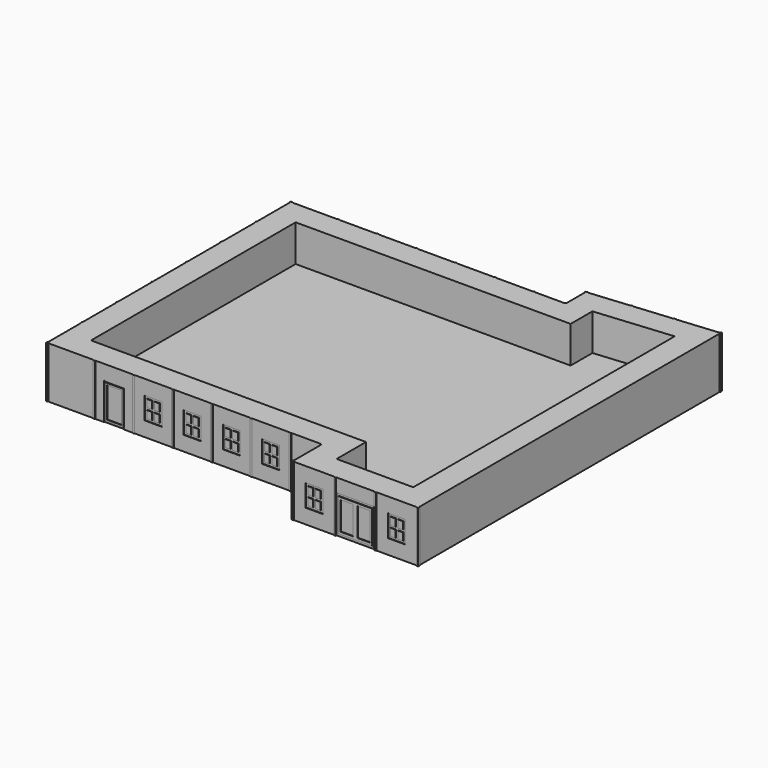
from build123d import *

# Parameters (mm, degrees)
F1_DEPTH  = 42
F3_DEPTH  = 30
F4_W      = 1.6
F4_H      = 42
F4_W_2    = 0.8
F6_W      = 1.6
F6_H      = 42
F13_DEPTH = 0.4
F5_W      = 0.8
F5_H      = 42
F5_W_2    = 1.6
F8_W      = 1.6
F8_H      = 42
F10_W     = 0.8
F10_H     = 42
F10_W_2   = 1.6
F14_DEPTH = 0.4
F7_W      = 0.4
F7_H      = 42
F7_W_2    = 1.2
F12_W     = 0.4368792842
F12_H     = 42
F12_W_2   = 1.1631207158
F12_W_3   = 0.3631207158
F15_DEPTH = 0.4
F9_W      = 1.6
F9_H      = 42
F9_W_2    = 0.8
F11_W     = 1.6
F11_H     = 42
F16_DEPTH = 0.4
F17_W     = 14.1428571429
F17_H     = 18
F17_W_2   = 4.1785714286
F17_H_2   = 6.1071428571
F18_W     = 14.1428571429
F18_H     = 18
F18_W_2   = 4.1785714286
F18_H_2   = 6.1071428571
F19_W     = 14.1428571429
F19_H     = 18
F19_W_2   = 4.1785714286
F19_H_2   = 6.1071428571
F20_DEPTH = 0.5
F21_W     = 17
F21_H     = 30
F21_W_2   = 15
F21_H_2   = 28
F21_W_3   = 12
F21_H_3   = 25
F22_DEPTH = 0.5
F23_W     = 31.4
F23_H     = 31
F23_W_2   = 27.4
F23_H_2   = 27
F23_W_3   = 10
F23_H_3   = 23
F24_DEPTH = 0.5
F25_W     = 14.1428571429
F25_H     = 18
F25_W_2   = 4.1785714286
F25_H_2   = 6.1071428571
F26_W     = 30.4
F26_H     = 31
F26_W_2   = 26.4
F26_H_2   = 27
F26_W_3   = 10
F26_H_3   = 23
F27_DEPTH = 0.5
F28_W     = 4.1785714286
F28_H     = 6.1071428571
F28_W_2   = 14.1428571429
F28_H_2   = 18
F29_DEPTH = 0.5


# Not quite as in the source:
# - a feature names something its author has since deleted; it is built from what else it names


with BuildPart() as f1:
    # F0 (on Top) → F1 (new body)
    with BuildSketch(Plane.XY):
        Polygon((-327.3, 108.1424002851), (-327.3, -140.8575997149), (-102.6, -140.8575997149), (-102.6, -170.8575997149), (0, -170.8575997149), (0, -140.8575997149), (0, 108.1424002851), (0, 138.1424002851), (-102.6, 128.6424002851), (-102.6, 108.1424002851), align=None)
    extrude(amount=F1_DEPTH)

    # F2 (on face) → F3 (cut)
    with BuildSketch(Plane.XY.offset(42)):
        Polygon((-20, 88.1424002851), (-20, 116.2049975252), (-82.6, 110.4087012289), (-82.6, 88.1424002851), (-307.3, 88.1424002851), (-307.3, -120.8575997149), (-82.6, -120.8575997149), (-82.6, -150.8575997149), (-20, -150.8575997149), (-20, -120.8575997149), align=None)
    extrude(amount=-F3_DEPTH, mode=Mode.SUBTRACT)

    # F4 (on face) + F6 (on face) → F13 (join)
    with BuildSketch(Plane.XZ.offset(140.8575997149)):
        with Locations((-288.375, 21)):
            Rectangle(F4_W, F4_H)
        with Locations((-256.375, 21)):
            Rectangle(F4_W, F4_H)
        with Locations((-224.375, 21)):
            Rectangle(F4_W, F4_H)
        with Locations((-192.375, 21)):
            Rectangle(F4_W, F4_H)
        with Locations((-160.375, 21)):
            Rectangle(F4_W, F4_H)
        with Locations((-128.375, 21)):
            Rectangle(F4_W, F4_H)
        with Locations((-103, 21)):
            Rectangle(F4_W_2, F4_H)
        with Locations((-326.9, 21)):
            Rectangle(F4_W, F4_H)
    with BuildSketch(Plane.XZ.offset(170.8575997149)):
        with Locations((-102.2, 21)):
            Rectangle(F6_W, F6_H)
        with Locations((-0.4, 21)):
            Rectangle(F6_W, F6_H)
        with Locations((-34.8, 21)):
            Rectangle(F6_W, F6_H)
        with Locations((-67.8, 21)):
            Rectangle(F6_W, F6_H)
    extrude(amount=F13_DEPTH)

    # F5 (on face) + F8 (on face) + F10 (on face) → F14 (join)
    with BuildSketch(Plane(origin=(-102.6, 0, 0), x_dir=(0, -1, 0), z_dir=(-1, 0, 0))):
        with Locations((141.2575997149, 21)):
            Rectangle(F5_W, F5_H)
        with Locations((170.4575997149, 21)):
            Rectangle(F5_W_2, F5_H)
    with BuildSketch(Plane(origin=(-327.3, 0, 0), x_dir=(0, -1, 0), z_dir=(-1, 0, 0))):
        with Locations((-108.0424002851, 21)):
            Rectangle(F8_W, F8_H)
        with Locations((-72.5424002851, 21)):
            Rectangle(F8_W, F8_H)
        with Locations((-37.0424002851, 21)):
            Rectangle(F8_W, F8_H)
        with Locations((-1.5424002851, 21)):
            Rectangle(F8_W, F8_H)
        with Locations((33.9575997149, 21)):
            Rectangle(F8_W, F8_H)
        with Locations((69.4575997149, 21)):
            Rectangle(F8_W, F8_H)
        with Locations((104.9575997149, 21)):
            Rectangle(F8_W, F8_H)
        with Locations((140.4575997149, 21)):
            Rectangle(F8_W, F8_H)
    with BuildSketch(Plane(origin=(-102.6, 0, 0), x_dir=(0, -1, 0), z_dir=(-1, 0, 0))):
        with Locations((-108.5424002851, 21)):
            Rectangle(F10_W, F10_H)
        with Locations((-128.2424002851, 21)):
            Rectangle(F10_W_2, F10_H)
    extrude(amount=F14_DEPTH)

    # F7 (on face) + F12 (on face) → F15 (join)
    with BuildSketch(Plane.YZ):
        with Locations((-171.0575997149, 21)):
            Rectangle(F7_W, F7_H)
        with Locations((-170.2575997149, 21)):
            Rectangle(F7_W_2, F7_H)
        with Locations((-171.4575997149, 21)):
            Rectangle(F7_W, F7_H)
    with BuildSketch(Plane.YZ):
        with Locations((138.3608399273, 21)):
            Rectangle(F12_W, F12_H)
        with Locations((137.5608399273, 21)):
            Rectangle(F12_W_2, F12_H)
        with Locations((138.7608399273, 21)):
            Rectangle(F12_W_3, F12_H)
    extrude(amount=F15_DEPTH)

    # F9 (on face) + F11 (on face) → F16 (join)
    with BuildSketch(Plane(origin=(0, 108.1424002851, 0), x_dir=(-1, 0, 0), z_dir=(0, 1, 0))):
        with Locations((288.375, 21)):
            Rectangle(F9_W, F9_H)
        with Locations((256.375, 21)):
            Rectangle(F9_W, F9_H)
        with Locations((224.375, 21)):
            Rectangle(F9_W, F9_H)
        with Locations((192.375, 21)):
            Rectangle(F9_W, F9_H)
        with Locations((160.375, 21)):
            Rectangle(F9_W, F9_H)
        with Locations((128.375, 21)):
            Rectangle(F9_W, F9_H)
        with Locations((103, 21)):
            Rectangle(F9_W_2, F9_H)
        with Locations((326.9, 21)):
            Rectangle(F9_W, F9_H)
    with BuildSketch(Plane(origin=(-12.6822332802, 136.9681194259, 0), x_dir=(-0.9957406741, -0.0921982106, 0), z_dir=(-0.0921982106, 0.9957406741, 0))):
        with Locations((-12.3364821089, 21)):
            Rectangle(F11_W, F11_H)
        with Locations((89.8655147654, 21)):
            Rectangle(F11_W, F11_H)
        with Locations((22.2829559704, 21)):
            Rectangle(F11_W, F11_H)
        with Locations((55.2829559704, 21)):
            Rectangle(F11_W, F11_H)
    extrude(amount=F16_DEPTH, dir=(0, 1, 0))

    # F17 (on face) + F18 (on face) + F19 (on face) → F20 (cut)
    with BuildSketch(Plane.XZ.offset(170.8575997149)):
        with Locations((-85.0000714286, 21)):
            Rectangle(F17_W, F17_H)
        with Locations((-88.0536428571, 16.9821428571)):
            Rectangle(F17_W_2, F17_H_2, mode=Mode.SUBTRACT)
        with Locations((-81.9465, 16.9821428571)):
            Rectangle(F17_W_2, F17_H_2, mode=Mode.SUBTRACT)
        with Locations((-88.0536428571, 25.0178571429)):
            Rectangle(F17_W_2, F17_H_2, mode=Mode.SUBTRACT)
        with Locations((-81.9465, 25.0178571429)):
            Rectangle(F17_W_2, F17_H_2, mode=Mode.SUBTRACT)
    with BuildSketch(Plane.XZ.offset(170.8575997149)):
        with Locations((-17.6000714286, 21)):
            Rectangle(F18_W, F18_H)
        with Locations((-20.6536428571, 16.9821428571)):
            Rectangle(F18_W_2, F18_H_2, mode=Mode.SUBTRACT)
        with Locations((-14.5465, 16.9821428571)):
            Rectangle(F18_W_2, F18_H_2, mode=Mode.SUBTRACT)
        with Locations((-20.6536428571, 25.0178571429)):
            Rectangle(F18_W_2, F18_H_2, mode=Mode.SUBTRACT)
        with Locations((-14.5465, 25.0178571429)):
            Rectangle(F18_W_2, F18_H_2, mode=Mode.SUBTRACT)
    with BuildSketch(Plane.XZ.offset(140.8575997149)):
        with Locations((-208.5035714286, 21)):
            Rectangle(F19_W, F19_H)
        with Locations((-211.5571428571, 16.9821428571)):
            Rectangle(F19_W_2, F19_H_2, mode=Mode.SUBTRACT)
        with Locations((-205.45, 16.9821428571)):
            Rectangle(F19_W_2, F19_H_2, mode=Mode.SUBTRACT)
        with Locations((-211.5571428571, 25.0178571429)):
            Rectangle(F19_W_2, F19_H_2, mode=Mode.SUBTRACT)
        with Locations((-205.45, 25.0178571429)):
            Rectangle(F19_W_2, F19_H_2, mode=Mode.SUBTRACT)
    extrude(amount=-F20_DEPTH, mode=Mode.SUBTRACT)

    # F21 (on face) → F22 (cut)
    with BuildSketch(Plane.XZ.offset(140.8575997149)):
        with Locations((-272.375, 15)):
            Rectangle(F21_W, F21_H)
        with Locations((-272.375, 15)):
            Rectangle(F21_W_2, F21_H_2, mode=Mode.SUBTRACT)
        with Locations((-272.375, 15)):
            Rectangle(F21_W_3, F21_H_3)
    extrude(amount=-F22_DEPTH, mode=Mode.SUBTRACT)

    # F23 (on face) → F24 (cut)
    with BuildSketch(Plane.XZ.offset(170.8575997149)):
        with Locations((-51.3, 15.5)):
            Rectangle(F23_W, F23_H)
        with Locations((-51.3, 15.5)):
            Rectangle(F23_W_2, F23_H_2, mode=Mode.SUBTRACT)
        with Locations((-58.3882954717, 15.5)):
            Rectangle(F23_W_3, F23_H_3)
        with Locations((-44.3882938325, 15.5)):
            Rectangle(F23_W_3, F23_H_3)
    extrude(amount=-F24_DEPTH, mode=Mode.SUBTRACT)

    # F25 (on face) + F26 (on face) → F27 (cut)
    with BuildSketch(Plane(origin=(-12.6822332802, 136.9681194259, 0), x_dir=(-0.9957406741, -0.0921982106, 0), z_dir=(-0.0921982106, 0.9957406741, 0))):
        with Locations((38.0461481147, 21)):
            Rectangle(F25_W, F25_H)
        with Locations((34.9925766862, 16.9821428571)):
            Rectangle(F25_W_2, F25_H_2, mode=Mode.SUBTRACT)
        with Locations((41.0997195433, 16.9821428571)):
            Rectangle(F25_W_2, F25_H_2, mode=Mode.SUBTRACT)
        with Locations((34.9925766862, 25.0178571429)):
            Rectangle(F25_W_2, F25_H_2, mode=Mode.SUBTRACT)
        with Locations((41.0997195433, 25.0178571429)):
            Rectangle(F25_W_2, F25_H_2, mode=Mode.SUBTRACT)
        with Locations((5.0461481147, 21)):
            Rectangle(F25_W, F25_H)
        with Locations((1.9925766862, 16.9821428571)):
            Rectangle(F25_W_2, F25_H_2, mode=Mode.SUBTRACT)
        with Locations((8.0997195433, 16.9821428571)):
            Rectangle(F25_W_2, F25_H_2, mode=Mode.SUBTRACT)
        with Locations((1.9925766862, 25.0178571429)):
            Rectangle(F25_W_2, F25_H_2, mode=Mode.SUBTRACT)
        with Locations((8.0997195433, 25.0178571429)):
            Rectangle(F25_W_2, F25_H_2, mode=Mode.SUBTRACT)
        with Locations((72.4460052576, 21)):
            Rectangle(F25_W, F25_H)
        with Locations((69.392433829, 16.9821428571)):
            Rectangle(F25_W_2, F25_H_2, mode=Mode.SUBTRACT)
        with Locations((75.4995766862, 16.9821428571)):
            Rectangle(F25_W_2, F25_H_2, mode=Mode.SUBTRACT)
        with Locations((69.392433829, 25.0178571429)):
            Rectangle(F25_W_2, F25_H_2, mode=Mode.SUBTRACT)
        with Locations((75.4995766862, 25.0178571429)):
            Rectangle(F25_W_2, F25_H_2, mode=Mode.SUBTRACT)
    with BuildSketch(Plane(origin=(0, 108.1424002851, 0), x_dir=(-1, 0, 0), z_dir=(0, 1, 0))):
        with Locations((272.375, 15.5)):
            Rectangle(F26_W, F26_H)
        with Locations((272.375, 15.5)):
            Rectangle(F26_W_2, F26_H_2, mode=Mode.SUBTRACT)
        with Locations((265.7867045283, 15.5)):
            Rectangle(F26_W_3, F26_H_3)
        with Locations((279.7867061675, 15.5)):
            Rectangle(F26_W_3, F26_H_3)
    extrude(amount=-F27_DEPTH, dir=(-0.0921982106, 0.9957406741, 0), mode=Mode.SUBTRACT)

    # F28 (on face) → F29 (cut)
    with BuildSketch(Plane.XZ.offset(140.8575997149)):
        Polygon((-233.4321428571, 30), (-247.575, 30), (-247.575, 12), (-233.4321428571, 12), (-233.4321428571, 12.718715705), align=None)
        with Locations((-243.5571428571, 16.9821428571)):
            Rectangle(F28_W, F28_H, mode=Mode.SUBTRACT)
        with Locations((-237.45, 16.9821428571)):
            Rectangle(F28_W, F28_H, mode=Mode.SUBTRACT)
        with Locations((-243.5571428571, 25.0178571429)):
            Rectangle(F28_W, F28_H, mode=Mode.SUBTRACT)
        with Locations((-237.45, 25.0178571429)):
            Rectangle(F28_W, F28_H, mode=Mode.SUBTRACT)
        with Locations((-176.5035714286, 21)):
            Rectangle(F28_W_2, F28_H_2)
        with Locations((-179.5571428571, 16.9821428571)):
            Rectangle(F28_W, F28_H, mode=Mode.SUBTRACT)
        with Locations((-173.45, 16.9821428571)):
            Rectangle(F28_W, F28_H, mode=Mode.SUBTRACT)
        with Locations((-179.5571428571, 25.0178571429)):
            Rectangle(F28_W, F28_H, mode=Mode.SUBTRACT)
        with Locations((-173.45, 25.0178571429)):
            Rectangle(F28_W, F28_H, mode=Mode.SUBTRACT)
        Polygon((-137.4321428571, 30), (-151.575, 30), (-151.575, 12), (-137.4321428571, 12), (-137.4321428571, 18.3077804595), align=None)
        with Locations((-147.5571428571, 16.9821428571)):
            Rectangle(F28_W, F28_H, mode=Mode.SUBTRACT)
        with Locations((-141.45, 16.9821428571)):
            Rectangle(F28_W, F28_H, mode=Mode.SUBTRACT)
        with Locations((-147.5571428571, 25.0178571429)):
            Rectangle(F28_W, F28_H, mode=Mode.SUBTRACT)
        with Locations((-141.45, 25.0178571429)):
            Rectangle(F28_W, F28_H, mode=Mode.SUBTRACT)
    extrude(amount=-F29_DEPTH, mode=Mode.SUBTRACT)


solid = f1.part
